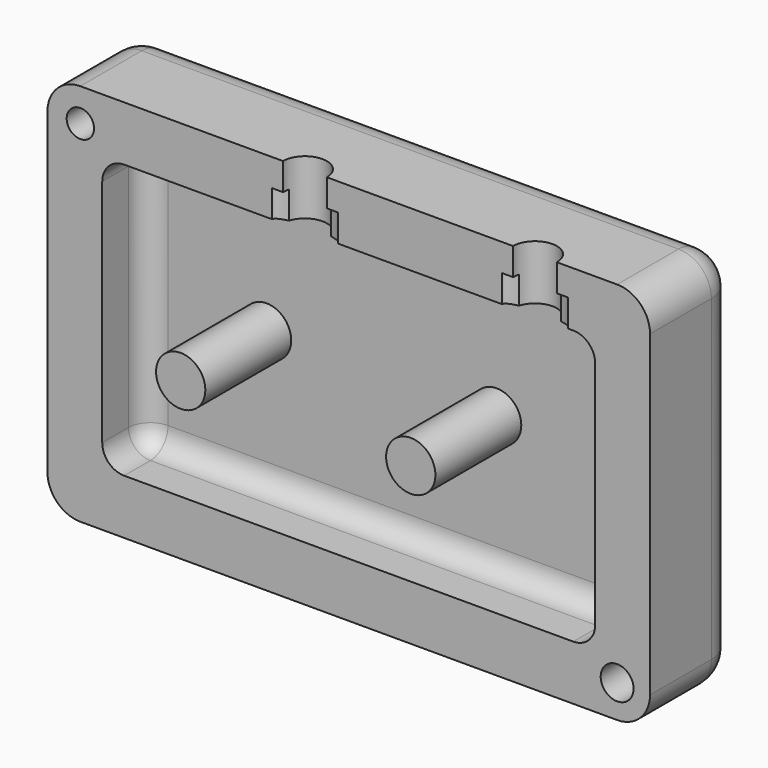
from build123d import *

# Parameters (mm, degrees)
F0_W      = 69.85
F0_H      = 44.45
F1_DEPTH  = 12.7
F2_T      = -6.35
F3_R      = 3.81
F4_R      = 2.54
F5_R      = 1.5875
F5_R_2    = 1.905
F6_DEPTH  = 5.08
F7_R      = 2.8575
F8_DEPTH  = 12.446
F9_R      = 2.54
F10_DEPTH = 6.35
F12_DEPTH = 3.175


# Not quite as in the source:
# - a feature names something its author has since deleted; it is built from what else it names


with BuildPart() as f1:
    # F0 (on Front) → F1 (new body)
    with BuildSketch(Plane.XZ):
        Rectangle(F0_W, F0_H)
    extrude(amount=-F1_DEPTH)

    # F2
    f2_openings = [f1.faces().sort_by_distance(p)[0] for p in [
        (0, 0, 0),
    ]]
    offset(amount=F2_T, openings=f2_openings)

    # F3
    f3_edges = [f1.edges().sort_by_distance(p)[0] for p in [
        (34.925, 6.35, -22.225),
        (34.925, 12.7, 0),
        (0, 12.7, -22.225),
        (-34.925, 12.7, 0),
        (0, 12.7, 22.225),
        (-34.925, 6.35, 22.225),
        (34.925, 6.35, 22.225),
        (-34.925, 6.35, -22.225),
    ]]
    fillet(f3_edges, radius=F3_R)

    # F4
    f4_edges = [f1.edges().sort_by_distance(p)[0] for p in [
        (-28.575, 6.35, 0),
        (0, 6.35, -15.875),
        (28.575, 6.35, 0),
        (0, 6.35, 15.875),
        (-28.575, 3.175, -15.875),
        (28.575, 3.175, -15.875),
        (28.575, 3.175, 15.875),
        (-28.575, 3.175, 15.875),
    ]]
    fillet(f4_edges, radius=F4_R)

    # F5 (on face) → F6 (cut)
    with BuildSketch(Plane.XZ):
        with Locations((-31.115, 18.415)):
            Circle(F5_R)
        with Locations((31.115, -18.415)):
            Circle(F5_R_2)
    extrude(amount=-F6_DEPTH, mode=Mode.SUBTRACT)

    # F7 (on face) → F8 (join)
    with BuildSketch(Plane.XZ.offset(-6.35)):
        with Locations((-14.605, 0)):
            Circle(F7_R)
        with Locations((12.065, 0)):
            Circle(F7_R)
    extrude(amount=F8_DEPTH)

    # F9 (on face) → F10 (cut, through all)
    with BuildSketch(Plane.XY.offset(22.225)):
        with Locations((-5.08, 0)):
            Circle(F9_R)
        with Locations((21.59, 0)):
            Circle(F9_R)
    extrude(amount=-F10_DEPTH, mode=Mode.SUBTRACT)

    # F11 (on face) → F12 (cut)
    with BuildSketch(Plane(origin=(0, 0, 15.875), x_dir=(1, 0, 0), z_dir=(0, 0, -1))):
        with BuildLine():
            add(Edge.make_bspline(
                [(-8.89, 0), (-8.89, -1.6497783942), (-3.175, -0.8248891971), (2.54, 0), (-3.175, 0.8248891971), (-8.89, 1.6497783942), (-8.89, 0)],
                knots=[0, 0, 0, 2.0943951024, 2.0943951024, 4.1887902048, 4.1887902048, 6.2831853072, 6.2831853072, 6.2831853072], degree=2, weights=[1, 0.5, 1, 0.5, 1, 0.5, 1]))
        make_face()
        with BuildLine():
            add(Edge.make_bspline(
                [(17.78, 0), (17.78, -1.6497783942), (23.495, -0.8248891971), (29.21, 0), (23.495, 0.8248891971), (17.78, 1.6497783942), (17.78, 0)],
                knots=[0, 0, 0, 2.0943951024, 2.0943951024, 4.1887902048, 4.1887902048, 6.2831853072, 6.2831853072, 6.2831853072], degree=2, weights=[1, 0.5, 1, 0.5, 1, 0.5, 1]))
        make_face()
    extrude(amount=-F12_DEPTH, mode=Mode.SUBTRACT)


solid = f1.part
